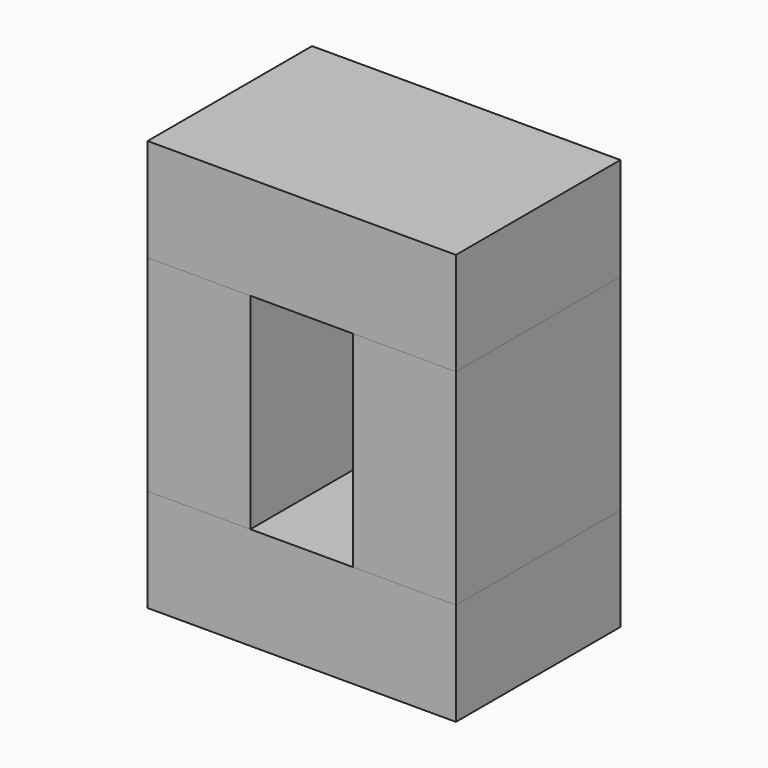
from build123d import *

# Parameters (mm, degrees)
F0_W     = 50.8
F0_H     = 101.6
F1_DEPTH = 101.6
F2_DEPTH = 101.6
F3_DEPTH = 101.6


# Not quite as in the source:
# - ends of sketch curves that miss each other by under 0.0002 mm in the source are joined


with BuildPart() as f1:
    # F0 (on Front) → F1 (new body)
    with BuildSketch(Plane.XZ):
        with Locations((50.8, 0)):
            Rectangle(F0_W, F0_H)
    extrude(amount=F1_DEPTH)


with BuildPart() as f1b:
    # F0 (on Front) → F1, piece 2 (new body)
    with BuildSketch(Plane.XZ):
        with Locations((-50.8, 0)):
            Rectangle(F0_W, F0_H)
    extrude(amount=F1_DEPTH)


with BuildPart() as f2:
    # F0 (on Front) → F2 (new body)
    with BuildSketch(Plane.XZ):
        Polygon((-76.2, 50.8), (-25.4, 50.8), (25.4, 50.8), (76.2, 50.8), (76.2000009418, 101.6), (-76.2, 101.6), align=None)
    extrude(amount=F2_DEPTH)


with BuildPart() as f3:
    # F0 (on Front) → F3 (new body)
    with BuildSketch(Plane.XZ):
        Polygon((25.4, -50.8), (-25.4, -50.8), (-76.2, -50.8), (-76.2, -101.6), (76.2, -101.6), (76.2, -50.8), align=None)
    extrude(amount=F3_DEPTH)


solid = Compound([f1.part, f1b.part, f2.part, f3.part])
